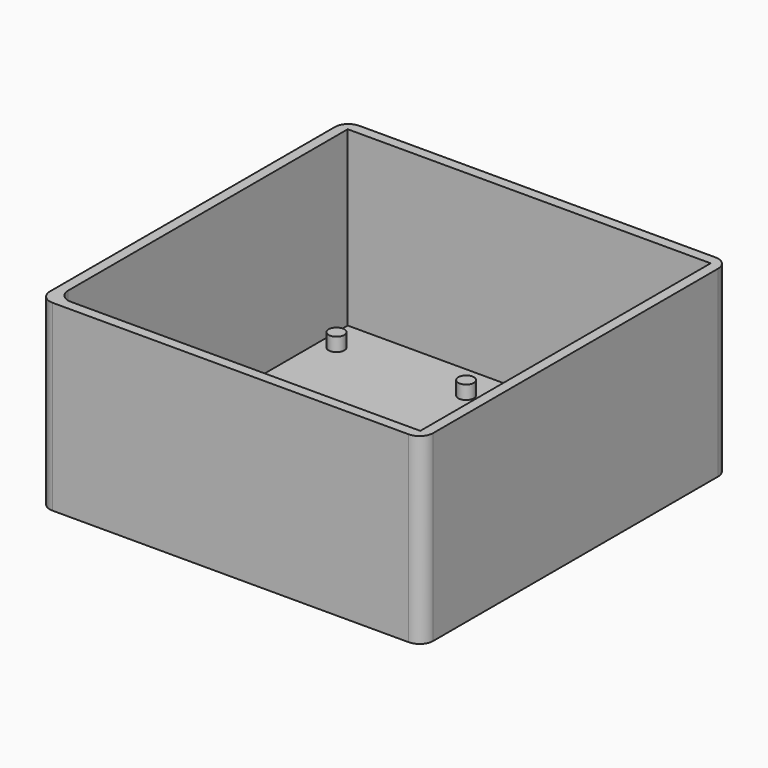
from build123d import *

# Parameters (mm, degrees)
F0_W     = 53.34
F0_H     = 53.34
F1_DEPTH = 25.4
F2_T     = 1.5
F3_R     = 1.27
F3_R_2   = 1.143
F4_DEPTH = 2
F5_R     = 2


# Not quite as in the source:
# - two fillets or chamfers of one size are made in one step


with BuildPart() as f1:
    # F0 (on Top) → F1 (new body)
    with BuildSketch(Plane.XY):
        Rectangle(F0_W, F0_H)
    extrude(amount=F1_DEPTH)

    # F2
    f2_openings = [f1.faces().sort_by_distance(p)[0] for p in [
        (0, 0, 25.4),
    ]]
    offset(amount=F2_T, openings=f2_openings, kind=Kind.INTERSECTION)

    # F3 (on face) → F4 (join)
    with BuildSketch(Plane.XY):
        with Locations((-23.63, -24.13)):
            Circle(F3_R)
        with Locations((-5.85, -24.13)):
            Circle(F3_R)
        with Locations((-24.253, 21.59)):
            Circle(F3_R_2)
        with Locations((-5.203, 21.59)):
            Circle(F3_R_2)
    extrude(amount=F4_DEPTH)

    # F5
    f5_edges = [f1.edges().sort_by_distance(p)[0] for p in [
        (-26.67, -26.67, 12.7),
        (28.17, -28.17, 11.95),
        (-28.17, -28.17, 11.95),
        (28.17, 28.17, 11.95),
        (-28.17, 28.17, 11.95),
    ]]
    fillet(f5_edges, radius=F5_R)


solid = f1.part
